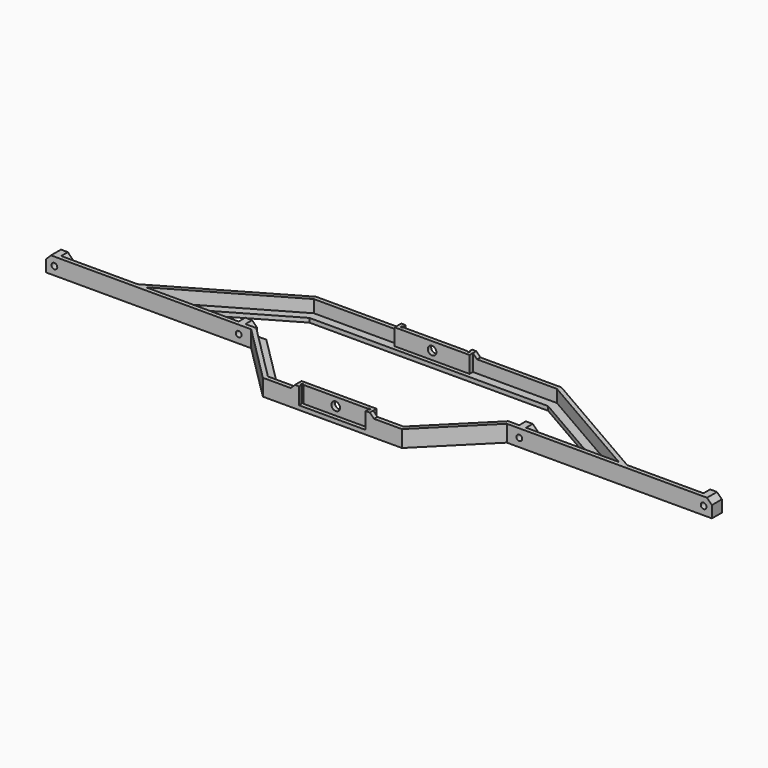
from build123d import *

# Parameters (mm, degrees)
F1_DEPTH  = 1.5875
F3_DEPTH  = 4.7625
F4_W      = 6.35
F4_H      = 6.35
F5_DEPTH  = 3.175
F6_SIZE   = 1.8598642
F7_W      = 28.575
F7_H      = 3.175
F8_DEPTH  = 1.5875
F9_W      = 25.4
F9_H      = 1.5875
F10_DEPTH = 6.35
F11_R     = 1.0922
F11_R_2   = 1.63322
F12_DEPTH = 25.4
F13_SIZE  = 1.58749
F14_R     = 0.396875
F15_DEPTH = 6.35
F16_R     = 1.63322
F17_DEPTH = 1.5875


# Not quite as in the source:
# - a fillet or chamfer is up to 0.001 mm smaller than in the source, because OpenCascade refuses the exact size


with BuildPart() as f1:
    # F0 (on Top) → F1 (new body)
    with BuildSketch(Plane.XY):
        Polygon((-87.87765, 22.225), (-127, 22.225), (-127, 17.4625), (-48.7553, 17.4625), (-26.5303, -4.7625), (26.5303, -4.7625), (48.7553, 17.4625), (127, 17.4625), (127, 22.225), (87.87765, 22.225), (46.7826079092, 45.9512336135), (-46.7826079092, 45.9512336135), align=None)
        Polygon((-24.5576079092, 0), (-46.7826079092, 22.225), (-78.35265, 22.225), (-45.5064998802, 41.1887336135), (45.5064998802, 41.1887336135), (78.35265, 22.225), (46.7826079092, 22.225), (24.5576079092, 0), align=None, mode=Mode.SUBTRACT)
    extrude(amount=F1_DEPTH)

    # F2 (on face) → F3 (join)
    with BuildSketch(Plane.XY.offset(1.5875)):
        Polygon((-127, 19.05), (-127, 17.4625), (-48.7553, 17.4625), (-26.5303, -4.7625), (26.5303, -4.7625), (48.7553, 17.4625), (127, 17.4625), (127, 19.05), (93.376911314, 19.05), (87.87765, 22.225), (46.7826079092, 45.9512336135), (-46.7826079092, 45.9512336135), (-87.87765, 22.225), (-93.376911314, 19.05), align=None)
        Polygon((90.201911314, 19.05), (48.0977359697, 19.05), (25.8727359697, -3.175), (14.2875, -3.175), (14.2875, -1.5875), (-14.2875, -1.5875), (-14.2875, -3.175), (-25.8727359697, -3.175), (-48.0977359697, 19.05), (-90.201911314, 19.05), (-46.3572385662, 44.3637336135), (-14.2875, 44.3637336135), (-14.2875, 42.7762336135), (14.2875, 42.7762336135), (14.2875, 44.3637336135), (46.3572385662, 44.3637336135), align=None, mode=Mode.SUBTRACT)
    extrude(amount=F3_DEPTH)

    # F4 (on face) → F5 (join, through all)
    with BuildSketch(Plane(origin=(0, 19.05, 0), x_dir=(-1, 0, 0), z_dir=(0, 1, 0))):
        with Locations((-53.5178, 3.175)):
            Rectangle(F4_W, F4_H)
        with Locations((-123.825, 3.175)):
            Rectangle(F4_W, F4_H)
        with Locations((123.825, 3.175)):
            Rectangle(F4_W, F4_H)
        with Locations((53.5178, 3.175)):
            Rectangle(F4_W, F4_H)
    extrude(amount=F5_DEPTH)

    # F6
    f6_edges = [f1.edges().sort_by_distance(p)[0] for p in [
        (-127, 19.84375, 6.35),
        (-120.65, 20.6375, 6.35),
        (-56.6928, 20.6375, 6.35),
        (-50.3428, 20.6375, 6.35),
        (50.3428, 20.6375, 6.35),
        (56.6928, 20.6375, 6.35),
        (120.65, 20.6375, 6.35),
        (127, 19.84375, 6.35),
    ]]
    chamfer(f6_edges, length=F6_SIZE)

    # F7 (on face) → F8 (join)
    with BuildSketch(Plane.XY.offset(6.35)):
        with Locations((0, -3.175)):
            Rectangle(F7_W, F7_H)
        with Locations((0, 44.3637336135)):
            Rectangle(F7_W, F7_H)
    extrude(amount=F8_DEPTH)

    # F9 (on face) → F10 (cut, through all)
    with BuildSketch(Plane.XY.offset(7.9375)):
        with Locations((0, -3.96875)):
            Rectangle(F9_W, F9_H)
        with Locations((0, 45.1574836135)):
            Rectangle(F9_W, F9_H)
    extrude(amount=-F10_DEPTH, mode=Mode.SUBTRACT)

    # F11 (on face) → F12 (cut, through all)
    with BuildSketch(Plane.XZ.offset(3.175)):
        with Locations((53.5178, 3.175)):
            Circle(F11_R)
        with Locations((123.825, 3.175)):
            Circle(F11_R)
        with Locations((-123.825, 3.175)):
            Circle(F11_R)
        with Locations((-53.5178, 3.175)):
            Circle(F11_R)
        with Locations((0, 4.7625)):
            Circle(F11_R_2)
    extrude(amount=-F12_DEPTH, mode=Mode.SUBTRACT)

    # F13 (size 1.5875 in the source; OpenCascade refuses exactly that, so slightly less here)
    f13_edges = [f1.edges().sort_by_distance(p)[0] for p in [
        (-14.2875, -3.96875, 6.35),
        (14.2875, -3.96875, 6.35),
        (-14.2875, 45.157484, 6.35),
        (14.2875, 45.157484, 6.35),
    ]]
    chamfer(f13_edges, length=F13_SIZE)

    # F14 (on face) → F15 (cut, through all)
    with BuildSketch(Plane.XY.offset(7.9375)):
        with Locations((-12.7, -3.175)):
            Circle(F14_R)
        with Locations((12.7, -3.175)):
            Circle(F14_R)
        with Locations((-12.7, 44.3637336135)):
            Circle(F14_R)
        with Locations((12.7, 44.3637336135)):
            Circle(F14_R)
    extrude(amount=-F15_DEPTH, mode=Mode.SUBTRACT)

    # F16 (on face) → F17 (cut, through all)
    with BuildSketch(Plane(origin=(0, 44.3637336135, 0), x_dir=(-1, 0, 0), z_dir=(0, 1, 0))):
        with Locations((0, 4.7625)):
            Circle(F16_R)
    extrude(amount=-F17_DEPTH, mode=Mode.SUBTRACT)


solid = f1.part
